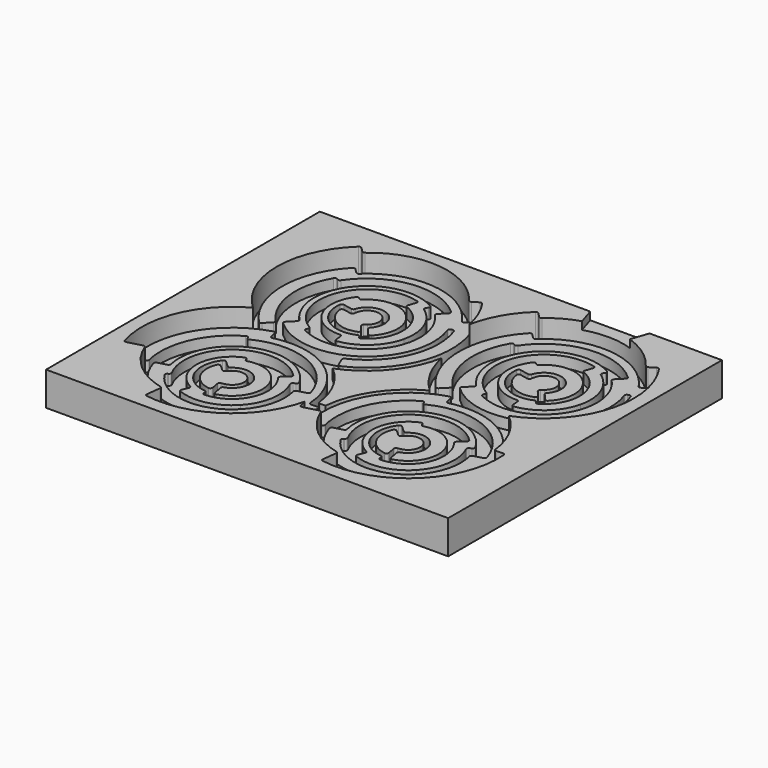
from build123d import *

# Parameters (mm, degrees)
F0_R      = 34.6612186842
F1_DEPTH  = 4
F3_DEPTH  = 4
F4_R      = 36.8076073985
F5_DEPTH  = 12.5
F6_R      = 0.8
F9_DEPTH  = 0.9
F12_ANGLE = 30
F17_DEPTH = 4.9
F19_DEPTH = 0.9
F21_DEPTH = 4
F22_DEPTH = 5
F23_W     = 151.6802990149
F23_H     = 129.0700121738
F24_DEPTH = 12.7
F28_DEPTH = 25
F29_ANGLE = -90


with BuildPart() as f1:
    # F0 (on Front) → F1 (new body)
    with BuildSketch(Plane.XZ):
        with Locations((0, -1.1545540765)):
            Circle(F0_R)
    extrude(amount=F1_DEPTH)

    # F2 (on Front) → F3 (cut, symmetric)
    with BuildSketch(Plane.XZ):
        with BuildLine():
            ThreePointArc((-9.746852, 16.453926), (16.0908880886, 11.1520903852), (14.142948, -15.151974))
            Line((14.142948, -15.151974), (17.678548, -18.687574))
            ThreePointArc((17.678548, -18.687574), (-2.9006382351, -25.7327450501), (-21.289452, -14.114274))
            Line((-21.289452, -14.114274), (-22.992652, -15.162574))
            add(Edge.make_bspline(
                [(-22.992652, -15.162574), (-29.546752, -4.514474), (-27.932352, 9.240626), (-19.091052, 18.082026)],
                knots=[0, 0, 0, 0, 1, 1, 1, 1], degree=3))
            Line((-19.091052, 18.082026), (-22.626552, 21.617526))
            ThreePointArc((-22.626552, 21.617526), (-32.0092911576, -1.009874), (-22.626552, -23.637274))
            Line((-22.626552, -23.637274), (-19.798152, -20.808874))
            add(Edge.make_bspline(
                [(3.066248, -28.841574), (-5.379252, -29.771774), (-13.790152, -26.816874), (-19.798152, -20.808874)],
                knots=[0, 0, 0, 0, 1, 1, 1, 1], degree=3))
            add(Edge.make_bspline(
                [(23.634348, -16.025174), (19.077948, -23.196674), (11.511748, -27.911374), (3.066248, -28.841574)],
                knots=[0, 0, 0, 0, 1, 1, 1, 1], degree=3))
            Line((23.634348, -16.025174), (27.010548, -18.170174))
            ThreePointArc((27.010548, -18.170174), (30.5166739714, 8.479008908), (12.516848, 28.440926))
            Line((12.516848, 28.440926), (10.561148, 23.839226))
            add(Edge.make_bspline(
                [(10.561148, 23.839226), (24.037748, 18.111926), (30.492748, 2.686326), (25.111548, -10.932174)],
                knots=[0, 0, 0, 0, 1, 1, 1, 1], degree=3))
            Line((25.111548, -10.932174), (23.251448, -10.197174))
            ThreePointArc((23.251448, -10.197174), (13.6562026484, 19.7938888186), (-17.676852, 16.667826))
            Line((-17.676852, 16.667826), (-14.141352, 13.132226))
            ThreePointArc((-14.141352, 13.132226), (-15.7811870352, -13.5538629713), (10.586548, -17.978674))
            Line((10.586548, -17.978674), (9.263348, -15.857574))
            add(Edge.make_bspline(
                [(17.037148, 2.992026), (18.751848, -4.307774), (15.625348, -11.888774), (9.263348, -15.857574)],
                knots=[0, 0, 0, 0, 1, 1, 1, 1], degree=3))
            add(Edge.make_bspline(
                [(1.683848, 16.409026), (9.147548, 15.687826), (15.322348, 10.291726), (17.037148, 2.992026)],
                knots=[0, 0, 0, 0, 1, 1, 1, 1], degree=3))
            Line((1.683848, 16.409026), (1.299148, 12.427526))
            add(Edge.make_bspline(
                [(-11.976452, 5.218726), (-9.435752, 10.104426), (-4.182152, 12.957126), (1.299148, 12.427526)],
                knots=[0, 0, 0, 0, 1, 1, 1, 1], degree=3))
            add(Edge.make_bspline(
                [(-10.254352, -9.789474), (-13.835652, -5.606174), (-14.517152, 0.333026), (-11.976452, 5.218726)],
                knots=[0, 0, 0, 0, 1, 1, 1, 1], degree=3))
            Line((-10.254352, -9.789474), (-8.735052, -8.488774))
            add(Edge.make_bspline(
                [(2.696448, -12.189474), (-1.506752, -13.202974), (-5.923152, -11.773274), (-8.735052, -8.488774)],
                knots=[0, 0, 0, 0, 1, 1, 1, 1], degree=3))
            add(Edge.make_bspline(
                [(11.185248, -3.685574), (10.179248, -7.890574), (6.899648, -11.175974), (2.696448, -12.189474)],
                knots=[0, 0, 0, 0, 1, 1, 1, 1], degree=3))
            add(Edge.make_bspline(
                [(7.464148, 7.739326), (10.753648, 4.933326), (12.191248, 0.519426), (11.185248, -3.685574)],
                knots=[0, 0, 0, 0, 1, 1, 1, 1], degree=3))
            Line((7.464148, 7.739326), (4.219248, 3.935326))
            add(Edge.make_bspline(
                [(4.219248, 3.935326), (6.383548, 2.089126), (7.095848, -0.949974), (5.977348, -3.565574)],
                knots=[0, 0, 0, 0, 1, 1, 1, 1], degree=3))
            add(Edge.make_bspline(
                [(5.977348, -3.565574), (4.858748, -6.181274), (2.169348, -7.765674), (-0.660652, -7.476174)],
                knots=[0, 0, 0, 0, 1, 1, 1, 1], degree=3))
            add(Edge.make_bspline(
                [(-0.660652, -7.476174), (-3.490652, -7.186674), (-5.803552, -5.090474), (-6.369352, -2.302574)],
                knots=[0, 0, 0, 0, 1, 1, 1, 1], degree=3))
            Line((-6.369352, -2.302574), (-11.269452, -3.296974))
            add(Edge.make_bspline(
                [(-11.269452, -3.296974), (-12.153552, 1.060026), (-10.447252, 5.536226), (-6.887252, 8.199026)],
                knots=[0, 0, 0, 0, 1, 1, 1, 1], degree=3))
            add(Edge.make_bspline(
                [(-6.887252, 8.199026), (-3.327152, 10.861926), (1.448748, 11.234226), (5.378448, 9.155326)],
                knots=[0, 0, 0, 0, 1, 1, 1, 1], degree=3))
            Line((5.378448, 9.155326), (6.313748, 10.923126))
            add(Edge.make_bspline(
                [(6.313748, 10.923126), (11.091748, 8.395426), (13.901348, 3.261426), (13.454648, -2.125474)],
                knots=[0, 0, 0, 0, 1, 1, 1, 1], degree=3))
            add(Edge.make_bspline(
                [(13.454648, -2.125474), (13.007948, -7.512374), (9.391148, -12.113474), (4.262048, -13.819674)],
                knots=[0, 0, 0, 0, 1, 1, 1, 1], degree=3))
            Line((4.262048, -13.819674), (5.709248, -18.170174))
            ThreePointArc((5.709248, -18.170174), (-16.5117148936, -8.2873575393), (-8.813452, 14.781626))
            Line((-8.813452, 14.781626), (-9.746852, 16.453926))
        make_face()
    extrude(amount=F3_DEPTH, both=True, mode=Mode.SUBTRACT)

    # F4 (on face) → F5 (cut, symmetric)
    with BuildSketch(Plane.XZ.offset(4)):
        with Locations((0.1748142323, -1.9060653497)):
            Circle(F4_R)
        with BuildLine():
            ThreePointArc((11.4376131926, 31.0148209034), (32.4264769291, 9.0728545636), (27.581184101, -20.9022255066))
            Line((27.581184101, -20.9022255066), (24.193680363, -18.7500439053))
            ThreePointArc((24.193680363, -18.7500439053), (3.3093339672, -31.0483867291), (-19.7510272312, -23.5901763545))
            Line((-19.7510272312, -23.5901763545), (-22.5838695578, -26.4230186825))
            ThreePointArc((-22.5838695578, -26.4230186825), (-33.9934209021, -1.009874), (-22.5838695578, 24.4032706825))
            Line((-22.5838695578, 24.4032706825), (-17.6768384376, 19.4962395624))
            ThreePointArc((-17.6768384376, 19.4962395624), (-5.1371917179, 25.4530784853), (8.7204829233, 24.6214996577))
            Line((8.7204829233, 24.6214996577), (11.4376131926, 31.0148209034))
        make_face(mode=Mode.SUBTRACT)
    extrude(amount=F5_DEPTH, both=True, mode=Mode.SUBTRACT)

    # F6
    f6_edges = [f1.edges().sort_by_distance(p)[0] for p in [
        (27.010548, -2, -18.170174),
        (14.142948, -2, -15.151974),
        (4.262048, -2, -13.819674),
        (-22.626552, -2, -23.637274),
        (-21.289452, -2, -14.114274),
        (-22.626552, -2, 21.617526),
        (-17.676852, -2, 16.667826),
        (-8.813452, -2, 14.781626),
        (5.378448, -2, 9.155326),
        (-10.254352, -2, -9.789474),
        (-6.369352, -2, -2.302574),
        (4.219248, -2, 3.935326),
        (10.561148, -2, 23.839226),
        (12.516848, -2, 28.440926),
        (10.586548, -2, -17.978674),
        (-19.091052, -2, 18.082026),
        (17.678548, -2, -18.687574),
        (23.251448, -2, -10.197174),
        (-14.141352, -2, 13.132226),
        (-9.746852, -2, 16.453926),
        (6.313748, -2, 10.923126),
        (-11.269452, -2, -3.296974),
        (7.464148, -2, 7.739326),
        (9.263348, -2, -15.857574),
        (25.111548, -2, -10.932174),
        (23.634348, -2, -16.025174),
        (-19.798152, -2, -20.808874),
        (1.299148, -2, 12.427526),
        (1.683848, -2, 16.409026),
        (5.709248, -2, -18.170174),
        (-8.735052, -2, -8.488774),
        (8.720483, -2, 24.6215),
        (-17.676838, -2, 19.49624),
        (-22.58387, -2, 24.403271),
        (11.437613, -2, 31.014821),
        (-19.751027, -2, -23.590176),
        (-22.58387, -2, -26.423019),
        (24.19368, -2, -18.750044),
        (27.581184, -2, -20.902226),
        (-22.992652, -2, -15.162574),
    ]]
    fillet(f6_edges, radius=F6_R)

    # F8 (on face) → F9 (join)
    with BuildSketch(Plane(origin=(0, 0, 0), x_dir=(-1, 0, 0), z_dir=(0, 1, 0))):
        with BuildLine():
            ThreePointArc((-12.1628911728, 30.7441200753), (-32.42647621, 9.0728568762), (-28.025070673, -20.2679705917))
            ThreePointArc((-28.025070673, -20.2679705917), (-27.5255767157, -20.6003491113), (-26.9354693925, -20.4919837998))
            Line((-26.9354693925, -20.4919837998), (-24.8278451869, -19.1529476278))
            ThreePointArc((-24.8278451869, -19.1529476278), (-24.2541917489, -19.0413788241), (-23.757728549, -19.3496808773))
            ThreePointArc((-23.757728549, -19.3496808773), (-3.3093364218, -31.0483864588), (19.1950155337, -24.0805606904))
            ThreePointArc((19.1950155337, -24.0805606904), (19.746680097, -23.8877008146), (20.2823011501, -24.1214502737))
            Line((20.2823011501, -24.1214502737), (22.0443264657, -25.8834755902))
            ThreePointArc((22.0443264657, -25.8834755902), (22.5956618868, -26.1176614534), (23.1550425876, -25.9034022721))
            ThreePointArc((23.1550425876, -25.9034022721), (33.9934209021, -1.0098739999), (23.1550425874, 23.8836542723))
            ThreePointArc((23.1550425874, 23.8836542723), (22.5956618868, 24.0979134535), (22.0443264657, 23.8637275905))
            Line((22.0443264657, 23.8637275905), (18.1870340017, 20.0064351265))
            ThreePointArc((18.1870340017, 20.0064351265), (17.6676162337, 19.7734596072), (17.1247702295, 19.9448965524))
            ThreePointArc((17.1247702295, 19.9448965524), (5.1371872176, 25.453079359), (-8.0406426711, 24.8309670505))
            ThreePointArc((-8.0406426711, 24.8309670505), (-8.6081965113, 24.8751220322), (-9.0026944769, 25.285534482))
            Line((-9.0026944769, 25.285534482), (-11.1383900878, 30.3107584392))
            ThreePointArc((-11.1383900878, 30.3107584392), (-11.5629936154, 30.7346437129), (-12.1628911728, 30.7441200753))
        make_face()
    extrude(amount=F9_DEPTH)


with BuildPart() as f10_1:
    # F10: copy of F1
    add(f1.part.moved(Location((66.7, 0, 0))))


with BuildPart() as f11_1:
    # F11: copy of F1
    add(f1.part.moved(Location((0, 0, 60.7))))


with BuildPart() as f11_1_1:
    # F12: moved
    add(f11_1.part.rotate(Axis((-0.660652, -2, 53.223826), (0, -1, 0)), F12_ANGLE))


with BuildPart() as f11_1_2:
    # F13: moved
    add(f11_1_1.part.moved(Location((-3.7, 0, -5.3))))


with BuildPart() as f14_1:
    # F14: copy of F11_1
    add(f11_1_2.part.moved(Location((66.4, 0, 0))))

    # F15: union F11_1, F10_1, F1
    add(f11_1_2.part)
    add(f10_1.part)
    add(f1.part)

    # F16 (on face) → F17 (join, through all)
    with BuildSketch(Plane.XZ.offset(4)):
        with BuildLine():
            ThreePointArc((74.7406426711, 24.8309670505), (75.3081965113, 24.8751220322), (75.7026944769, 25.285534482))
            Line((75.7026944769, 25.285534482), (77.5972127455, 29.7432758107))
            ThreePointArc((77.5972127455, 29.7432758107), (74.1386798608, 27.4897808861), (70.3998927938, 25.7401636831))
            ThreePointArc((70.3998927938, 25.7401636831), (72.5883814369, 25.372045076), (74.7406426711, 24.8309670505))
        make_face()
        with BuildLine():
            ThreePointArc((56.4699937083, 23.9489122844), (55.3770945219, 24.0925397154), (54.2903116821, 24.276823545))
            ThreePointArc((54.2903116821, 24.276823545), (53.716126218, 24.1680128152), (53.3691395087, 23.6977693189))
            Line((53.3691395087, 23.6977693189), (52.9824725775, 22.2547086848))
            ThreePointArc((52.9824725775, 22.2547086848), (54.6967354041, 23.1625316324), (56.4699937083, 23.9489122844))
        make_face()
        with BuildLine():
            ThreePointArc((49.5752297705, 19.9448965524), (50.2300614071, 20.4477343717), (50.8995001184, 20.9309549804))
            ThreePointArc((50.8995001184, 20.9309549804), (48.3439912436, 21.6979456057), (45.8564785099, 22.6629226148))
            Line((45.8564785099, 22.6629226148), (48.5129659983, 20.0064351265))
            ThreePointArc((48.5129659983, 20.0064351265), (49.0323837663, 19.7734596072), (49.5752297705, 19.9448965524))
        make_face()
        with BuildLine():
            ThreePointArc((3.9232754984, 25.7107627943), (5.9985966351, 25.3487272036), (8.0406426711, 24.8309670505))
            ThreePointArc((8.0406426711, 24.8309670505), (8.6081965113, 24.8751220322), (9.0026944769, 25.285534482))
            Line((9.0026944769, 25.285534482), (10.7591245405, 29.4183586492))
            ThreePointArc((10.7591245405, 29.4183586492), (7.4636825779, 27.3387345226), (3.9232754984, 25.7107627943))
        make_face()
        with BuildLine():
            ThreePointArc((-10.1624580024, 23.9759933269), (-11.1385809042, 24.1101761732), (-12.1096883179, 24.276823545))
            ThreePointArc((-12.1096883179, 24.276823545), (-12.683873782, 24.1680128152), (-13.0308604913, 23.6977693189))
            Line((-13.0308604913, 23.6977693189), (-13.3639695944, 22.4545892206))
            ThreePointArc((-13.3639695944, 22.4545892206), (-11.7874255611, 23.2662404192), (-10.1624580024, 23.9759933269))
        make_face()
        with BuildLine():
            ThreePointArc((-17.1247702295, 19.9448965524), (-16.4299133669, 20.4774817319), (-15.7186712618, 20.987979235))
            ThreePointArc((-15.7186712618, 20.987979235), (-18.441111423, 21.832792874), (-21.083236204, 22.9026373288))
            Line((-21.083236204, 22.9026373288), (-18.1870340017, 20.0064351265))
            ThreePointArc((-18.1870340017, 20.0064351265), (-17.6676162337, 19.7734596072), (-17.1247702295, 19.9448965524))
        make_face()
    extrude(amount=-F17_DEPTH)

    # F18 (on face) → F19 (join, through all)
    with BuildSketch(Plane(origin=(0, 0.9, 0), x_dir=(-1, 0, 0), z_dir=(0, 1, 0))):
        with BuildLine():
            ThreePointArc((-43.4678642949, 23.8116800848), (-36.9537938006, 15.4470378395), (-33.3321508048, 5.4828993263))
            ThreePointArc((-33.3321508048, 5.4828993263), (-26.0716647312, 20.7623231189), (-12.3583698918, 30.6679272956))
            ThreePointArc((-12.3583698918, 30.6679272956), (-19.3743604558, 39.2683246145), (-22.7230393134, 49.8502576867))
            ThreePointArc((-22.7230393134, 49.8502576867), (-22.9988380299, 50.3654866968), (-23.551420882, 50.5556919975))
            Line((-23.551420882, 50.5556919975), (-25.5525127339, 50.4708065494))
            ThreePointArc((-25.5525127339, 50.4708065494), (-31.1644356109, 34.892844834), (-43.4678642949, 23.8116800848))
        make_face()
    extrude(amount=-F19_DEPTH)

    # F20 (on face) → F21 (cut, through all)
    with BuildSketch(Plane.XZ.offset(4)):
        with BuildLine():
            Line((-11.1873683429, 51.7736616655), (-10.3926712745, 50.8745197141))
            ThreePointArc((-10.3926712745, 50.8745197141), (-3.1041609019, 51.6389526025), (-6.2035359316, 58.2797820324))
            Line((-6.2035359316, 58.2797820324), (-7.452363586, 58.5104483506))
            ThreePointArc((-7.452363586, 58.5104483506), (-7.9660800475, 58.8436130505), (-8.0937494226, 59.4424484626))
            Line((-8.0937494226, 59.4424484626), (-7.5646045507, 62.3072392755))
            ThreePointArc((-7.5646045507, 62.3072392755), (-7.7773324366, 63.0098291756), (-8.4733440578, 63.243182008))
            add(Edge.make_bspline(
                [(-15.7523914912, 57.5976488586), (-15.3901688204, 58.4426116153), (-14.4405638027, 59.9866168832), (-12.4655388269, 61.7890880588), (-10.3961035899, 62.8222758991), (-9.0049146534, 63.1611260664), (-8.4733440578, 63.243182008)],
                knots=[0, 0, 0, 0, 0.25, 0.5, 0.75, 0.8987834998, 0.8987834998, 0.8987834998, 0.8987834998], degree=3))
            add(Edge.make_bspline(
                [(-15.7855097532, 50.1888698789), (-16.0757336256, 50.8832167796), (-16.5246518545, 52.4629652799), (-16.5781074948, 55.0003837495), (-16.1146033138, 56.7527219988), (-15.7523914912, 57.5976488586)],
                knots=[0.2881145227, 0.2881145227, 0.2881145227, 0.2881145227, 0.5, 0.75, 1, 1, 1, 1], degree=3))
            ThreePointArc((-15.7855097532, 50.1888698789), (-15.2262958891, 49.7176490967), (-14.517595021, 49.897960635))
            Line((-14.517595021, 49.897960635), (-13.2158263955, 51.0485150148))
            Line((-13.2158263955, 51.0485150148), (-12.3165944818, 51.8432915954))
            ThreePointArc((-12.3165944818, 51.8432915954), (-11.7375605817, 52.0423470213), (-11.1873683429, 51.7736616655))
        make_face()
        with BuildLine():
            Line((55.2126315686, 51.7736617657), (56.0073287255, 50.8745197141))
            ThreePointArc((56.0073287255, 50.8745197141), (63.3028469135, 51.651386502), (60.1683771237, 58.2848777981))
            Line((60.1683771237, 58.2848777981), (59.0164081622, 58.4976537068))
            ThreePointArc((59.0164081622, 58.4976537068), (58.5026917007, 58.8308184067), (58.3750223256, 59.4296538188))
            Line((58.3750223256, 59.4296538188), (58.9085177872, 62.317998728))
            ThreePointArc((58.9085177872, 62.317998728), (58.6980512579, 63.0182500828), (58.0062122515, 63.2549078715))
            ThreePointArc((58.0062122515, 63.2549078715), (51.1104640961, 58.5321837796), (50.6148290437, 50.1889343307))
            ThreePointArc((50.6148290437, 50.1889343307), (51.1740618151, 49.7178644556), (51.8826719799, 49.8981967992))
            Line((51.8826719799, 49.8981967992), (54.0834054297, 51.8432916955))
            ThreePointArc((54.0834054297, 51.8432916955), (54.6624393298, 52.0423471215), (55.2126315686, 51.7736617657))
        make_face()
        with BuildLine():
            Line((-4.6478439712, -0.7287602108), (-4.4091870708, -1.9047886475))
            ThreePointArc((-4.4091870708, -1.9047886475), (2.2850645118, -4.887025533), (2.9213417152, 2.4137889704))
            Line((2.9213417152, 2.4137889704), (2.0083779174, 3.19256821))
            ThreePointArc((2.0083779174, 3.19256821), (1.7300687613, 3.7379555344), (1.9189215453, 4.3203969015))
            Line((1.9189215453, 4.3203969015), (3.8250558648, 6.5549603553))
            ThreePointArc((3.8250558648, 6.5549603553), (3.9929121812, 7.2666290822), (3.5120909206, 7.8175002425))
            ThreePointArc((3.5120909206, 7.8175002425), (-4.821164206, 7.1753752815), (-9.4220214768, 0.1977268349))
            ThreePointArc((-9.4220214768, 0.1977268349), (-9.1732466278, -0.4898480296), (-8.4694060518, -0.6879807213))
            Line((-8.4694060518, -0.6879807213), (-5.5909675292, -0.1038458533))
            ThreePointArc((-5.5909675292, -0.1038458533), (-4.9899817491, -0.2209757477), (-4.6478439712, -0.7287602108))
        make_face()
        with BuildLine():
            Line((62.0521560288, -0.7287602108), (62.2908129292, -1.9047886475))
            ThreePointArc((62.2908129292, -1.9047886475), (68.9850645118, -4.887025533), (69.6213417152, 2.4137889704))
            Line((69.6213417152, 2.4137889704), (68.7083779174, 3.19256821))
            ThreePointArc((68.7083779174, 3.19256821), (68.4300687613, 3.7379555344), (68.6189215453, 4.3203969015))
            Line((68.6189215453, 4.3203969015), (70.5250558648, 6.5549603553))
            ThreePointArc((70.5250558648, 6.5549603553), (70.6929121812, 7.2666290822), (70.2120909206, 7.8175002425))
            ThreePointArc((70.2120909206, 7.8175002425), (61.878835794, 7.1753752815), (57.2779785232, 0.1977268349))
            ThreePointArc((57.2779785232, 0.1977268349), (57.5267533722, -0.4898480296), (58.2305939482, -0.6879807213))
            Line((58.2305939482, -0.6879807213), (61.1090324708, -0.1038458533))
            ThreePointArc((61.1090324708, -0.1038458533), (61.7100182509, -0.2209757477), (62.0521560288, -0.7287602108))
        make_face()
    extrude(amount=-F21_DEPTH, mode=Mode.SUBTRACT)

    # F22 (add): a face of the model
    f22_faces = [f14_1.faces().sort_by_distance(p)[0] for p in [
        (29.9306129486, 0.9, 26.3552797861),
    ]]
    extrude(f22_faces, amount=F22_DEPTH)


with BuildPart() as f24:
    # F23 (on face) → F24 (new body)
    with BuildSketch(Plane(origin=(0, 5.9, 0), x_dir=(-1, 0, 0), z_dir=(0, 1, 0))):
        with Locations((-29.8232689666, 28.3089755943)):
            Rectangle(F23_W, F23_H)
    extrude(amount=-F24_DEPTH)

    # F25: cut F14_1
    add(f14_1.part, mode=Mode.SUBTRACT)

    # F27 (on offset) → F28 (cut)
    with BuildSketch(Plane(origin=(0, 3, 0), x_dir=(-1, 0, 0), z_dir=(0, 1, 0))):
        with BuildLine():
            Line((-55.9893287718, -36.2260304926), (-57.9687839973, -29.8838792687))
            ThreePointArc((-57.9687839973, -29.8838792687), (-67.0774355079, -31.2244710795), (-76.1566229517, -29.6970307022))
            Line((-76.1566229517, -29.6970307022), (-78.3425777495, -36.2260304926))
            Line((-78.3425777495, -36.2260304926), (-55.9893287718, -36.2260304926))
        make_face()
    extrude(amount=F28_DEPTH, mode=Mode.SUBTRACT)


with BuildPart() as f24_1:
    # F29: moved
    add(f24.part.rotate(Axis((29.8232689666, -6.8, -36.2260304926), (-1, 0, 0)), F29_ANGLE))


with BuildPart() as f24_2:
    # F30: moved
    add(f24_1.part.moved(Location((-29.822, 71.339, 36.225))))


solid = f24_2.part
